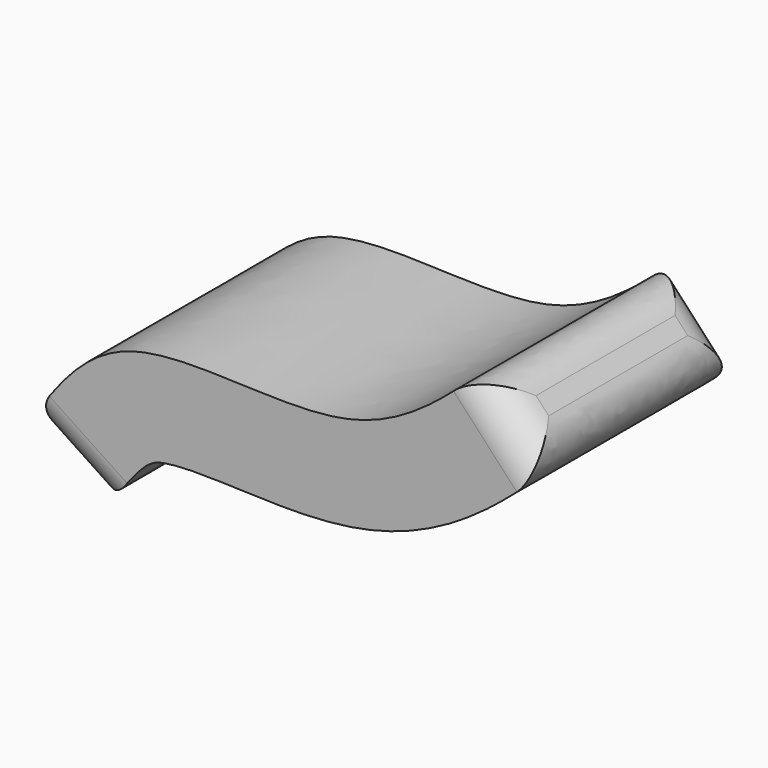
from build123d import *

# Parameters (mm, degrees)
F1_DEPTH = 50.8
F2_R     = 7.62


# Not quite as in the source:
# - the dataset's text gives a spline's control points without its knots; the knots are read off the source's solid


with BuildPart() as f1:
    # F0 (on Front) → F1 (new body)
    with BuildSketch(Plane.XZ):
        with BuildLine():
            add(Edge.make_bspline(
                [(-51.0408617556, 0), (-45.5275415756, 8.3222117367), (-33.1728131458, 26.9713492051), (15.9381703449, 15.4898879926), (33.4564530938, 31.6988813075), (41.5815524757, 39.2167232931)],
                knots=[0, 0, 0, 0, 0.3017270247, 0.6761362172, 1, 1, 1, 1], degree=3))
            Line((-51.0408617556, 0), (-35.1597019204, -10.5209915069))
            add(Edge.make_bspline(
                [(-35.1597019204, -10.5209915069), (-34.0176679526, -8.7971212834), (-32.4436828955, -6.4289476549), (-30.5673961608, -3.844107074), (-29.2783594821, -2.2206757706), (-28.1224556356, -0.9303565603), (-27.1210118733, 0.0294254181), (-26.427429255, 0.5807963747), (-25.9491520867, 0.9059703006), (-25.6216745244, 1.1026978633), (-25.3148685346, 1.2632261503), (-25.0156656107, 1.3975091183), (-24.7534837721, 1.4958188175), (-24.53491931, 1.5662690462), (-24.3240544361, 1.6271387901), (-24.0660733701, 1.6933193952), (-23.6603436757, 1.7855318353), (-22.791571975, 1.9500019347), (-21.1236299266, 2.157569393), (-18.5454924397, 2.3020094371), (-15.4940252899, 2.3309953909), (-12.0557374475, 2.2624077187), (-8.2992802909, 2.131996953), (-4.2762269139, 1.9869386104), (-0.0220731549, 1.8837160535), (3.6990437901, 1.8878531223), (6.7794439764, 1.9860069299), (9.1424813896, 2.1194163727), (11.5593646659, 2.326335526), (14.0327137076, 2.6230416895), (16.1394099163, 2.959867021), (17.8584301073, 3.295613243), (19.1296511182, 3.5752662629), (20.3839486951, 3.8818598634), (22.0321693162, 4.3253575728), (24.8512388207, 5.1890841749), (28.6793925567, 6.6518174582), (32.9317814942, 8.6951058623), (36.8413517827, 10.9454044623), (40.4245860953, 13.3273576493), (44.8048318302, 16.5921251267), (49.6210716705, 20.6981173805), (52.9512719821, 23.7831411529), (54.5192729081, 25.2339521081)],
                knots=[0, 0, 0, 0, 0.0625, 0.09375, 0.125, 0.15625, 0.1875, 0.21875, 0.234375, 0.25, 0.265625, 0.28125, 0.296875, 0.3046875, 0.3125, 0.3203125, 0.328125, 0.34375, 0.375, 0.40625, 0.4375, 0.46875, 0.5, 0.53125, 0.5625, 0.59375, 0.609375, 0.625, 0.640625, 0.65625, 0.671875, 0.6796875, 0.6875, 0.6953125, 0.703125, 0.71875, 0.75, 0.78125, 0.8125, 0.84375, 0.875, 0.9375, 1, 1, 1, 1], degree=3))
            Line((54.5192729081, 25.2339521081), (41.5815524757, 39.2167232931))
        make_face()
    extrude(amount=F1_DEPTH)

    # F2
    f2_edges = [f1.edges().sort_by_distance(p)[0] for p in [
        (41.581552, -25.4, 39.216723),
        (54.519273, -25.4, 25.233952),
        (48.050413, 0, 32.225338),
        (48.050413, -50.8, 32.225338),
        (-35.159702, -25.4, -10.520992),
        (-51.040862, -25.4, 0),
        (-43.100282, 0, -5.260496),
        (-43.100282, -50.8, -5.260496),
    ]]
    fillet(f2_edges, radius=F2_R)


solid = f1.part
